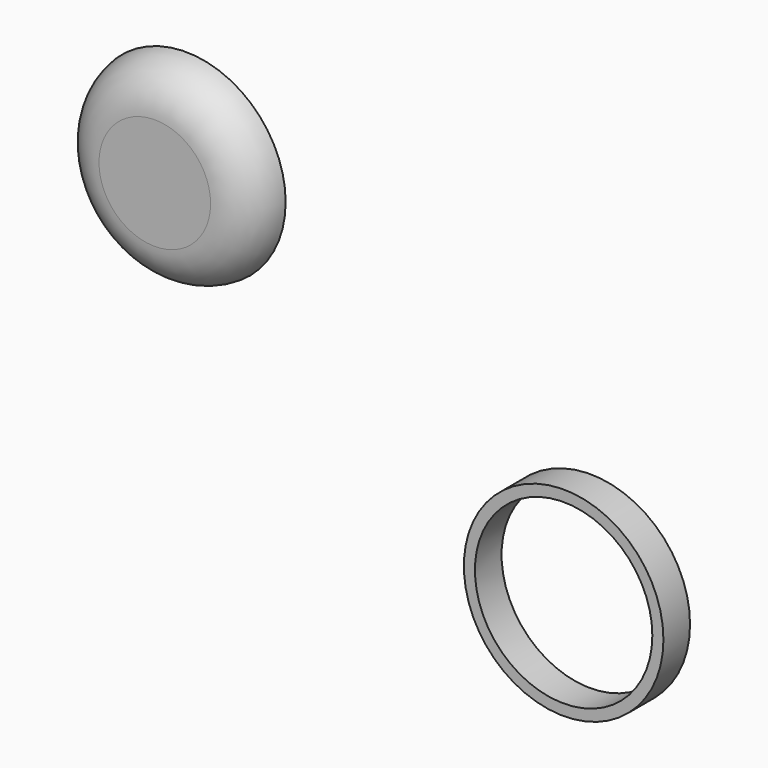
from build123d import *

# Parameters (mm, degrees)
F0_R     = 11.43
F0_R_2   = 10.16
F1_DEPTH = 3.81
F2_R     = 11.43
F3_DEPTH = 4.445


# Not quite as in the source:
# - a fillet or chamfer that OpenCascade refuses, or shapes differently, is made with other operations: its cross-section is extruded or revolved along the edge and cut away or added


with BuildPart() as f1:
    # F0 (on Front) → F1 (new body)
    with BuildSketch(Plane.XZ):
        Circle(F0_R)
        Circle(F0_R_2, mode=Mode.SUBTRACT)
    extrude(amount=F1_DEPTH)


with BuildPart() as f3:
    # F2 (on Front) → F3 (new body)
    with BuildSketch(Plane.XZ):
        with Locations((-46.3215783238, 27.5122094899)):
            Circle(F2_R)
    extrude(amount=F3_DEPTH)

    # F4: fillet of radius 5.08 on 1 edges, made by hand

    # F4_s1 → F4_t2 (revolve, cut)
    with BuildSketch(Plane.XY.offset(27.5122094899)):
        with BuildLine():
            ThreePointArc((-34.8915783238, 0), (-36.5716304064, -3.175), (-39.9317345714, -4.445))
            Line((-39.9317345714, -4.445), (-34.8915783238, -4.445))
            Line((-34.8915783238, -4.445), (-34.8915783238, 0))
        make_face()
    revolve(axis=Axis((-46.3215783238, -4.445, 27.5122094899), (0, -1, 0)), mode=Mode.SUBTRACT)


solid = Compound([f1.part, f3.part])
